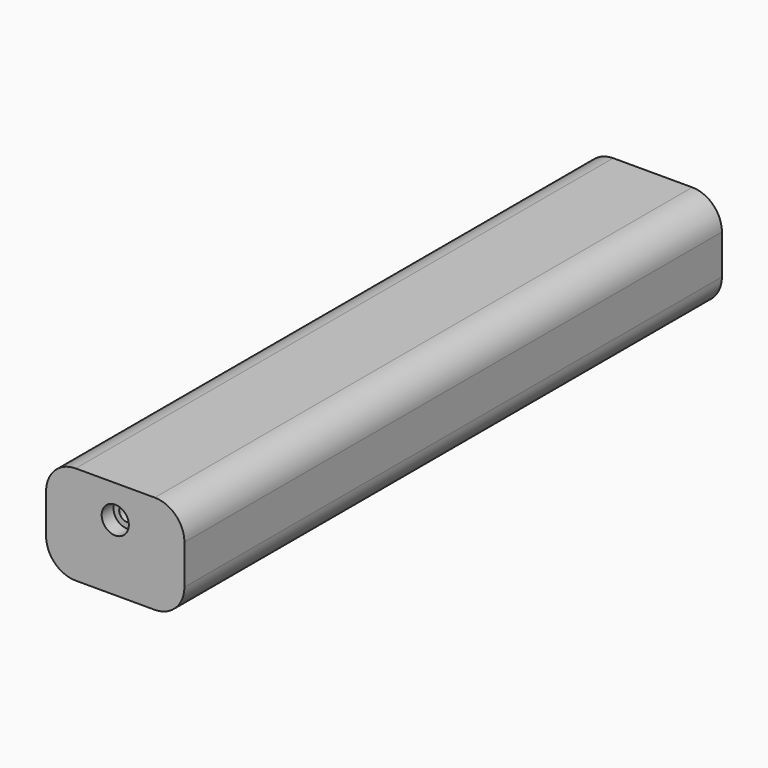
from build123d import *

# Parameters (mm, degrees)
F0_W        = 28
F0_H        = 20
F1_DEPTH    = 68
F3_DEPTH    = 15
F2_W        = 24
F2_H        = 100
F4_DEPTH    = 18
F5_T1_DEPTH = 166
F6_R        = 1.6
F7_DEPTH    = 140
F6_R_2      = 2.75
F8_DEPTH    = 3
F9_R        = 2.75
F9_R_2      = 1.6
F10_DEPTH   = 3


# Not quite as in the source:
# - a fillet or chamfer that OpenCascade refuses, or shapes differently, is made with other operations: its cross-section is extruded or revolved along the edge and cut away or added


with BuildPart() as f1:
    # F0 (on Front) → F1 (new body, symmetric)
    with BuildSketch(Plane.XZ):
        Rectangle(F0_W, F0_H)
    extrude(amount=F1_DEPTH, both=True)

    # F2 (on face) → F3 (cut)
    with BuildSketch(Plane(origin=(0, 0, -10), x_dir=(1, 0, 0), z_dir=(0, 0, -1))):
        Polygon((12, 62), (-12, 62), (-12, 53.5), (-10.3, 53.5), (-10.3, 60.3), (10.3, 60.3), (10.3, 53.5), (12, 53.5), align=None)
        Polygon((-12, -53.5), (-12, -62), (12, -62), (12, -53.5), (10.3, -53.5), (10.3, -60.3), (-10.3, -60.3), (-10.3, -53.5), align=None)
    extrude(amount=-F3_DEPTH, mode=Mode.SUBTRACT)

    # F2 (on face) → F4 (cut)
    with BuildSketch(Plane(origin=(0, 0, -10), x_dir=(1, 0, 0), z_dir=(0, 0, -1))):
        Rectangle(F2_W, F2_H)
    extrude(amount=-F4_DEPTH, mode=Mode.SUBTRACT)

    # F5: fillet of radius 6 on 4 edges, made by hand

    # F5_s2 → F5_t1 (cut)
    with BuildSketch(Plane.XZ.offset(-83)):
        with BuildLine():
            ThreePointArc((-8, 10), (-12.2426406871, 8.2426406871), (-14, 4))
            Line((-14, 4), (-14, 10))
            Line((-14, 10), (-8, 10))
        make_face()
        with BuildLine():
            ThreePointArc((8, 10), (12.2426406871, 8.2426406871), (14, 4))
            Line((14, 4), (14, 10))
            Line((14, 10), (8, 10))
        make_face()
        with BuildLine():
            ThreePointArc((14, -4), (12.2426406871, -8.2426406871), (8, -10))
            Line((8, -10), (14, -10))
            Line((14, -10), (14, -4))
        make_face()
        with BuildLine():
            ThreePointArc((-14, -4), (-12.2426406871, -8.2426406871), (-8, -10))
            Line((-8, -10), (-14, -10))
            Line((-14, -10), (-14, -4))
        make_face()
    extrude(amount=F5_T1_DEPTH, mode=Mode.SUBTRACT)

    # F6 (on face) → F7 (cut)
    with BuildSketch(Plane(origin=(0, 68, 0), x_dir=(-1, 0, 0), z_dir=(0, 1, 0))):
        with Locations((0, 3.4)):
            Circle(F6_R)
    extrude(amount=-F7_DEPTH, mode=Mode.SUBTRACT)

    # F6 (on face) → F8 (cut)
    with BuildSketch(Plane(origin=(0, 68, 0), x_dir=(-1, 0, 0), z_dir=(0, 1, 0))):
        with Locations((0, 3.4)):
            Circle(F6_R_2)
        with Locations((0, 3.4)):
            Circle(F6_R, mode=Mode.SUBTRACT)
    extrude(amount=-F8_DEPTH, mode=Mode.SUBTRACT)

    # F9 (on face) → F10 (cut)
    with BuildSketch(Plane.XZ.offset(68)):
        with Locations((0, 3.4)):
            Circle(F9_R)
        with Locations((0, 3.4)):
            Circle(F9_R_2, mode=Mode.SUBTRACT)
    extrude(amount=-F10_DEPTH, mode=Mode.SUBTRACT)


solid = f1.part
